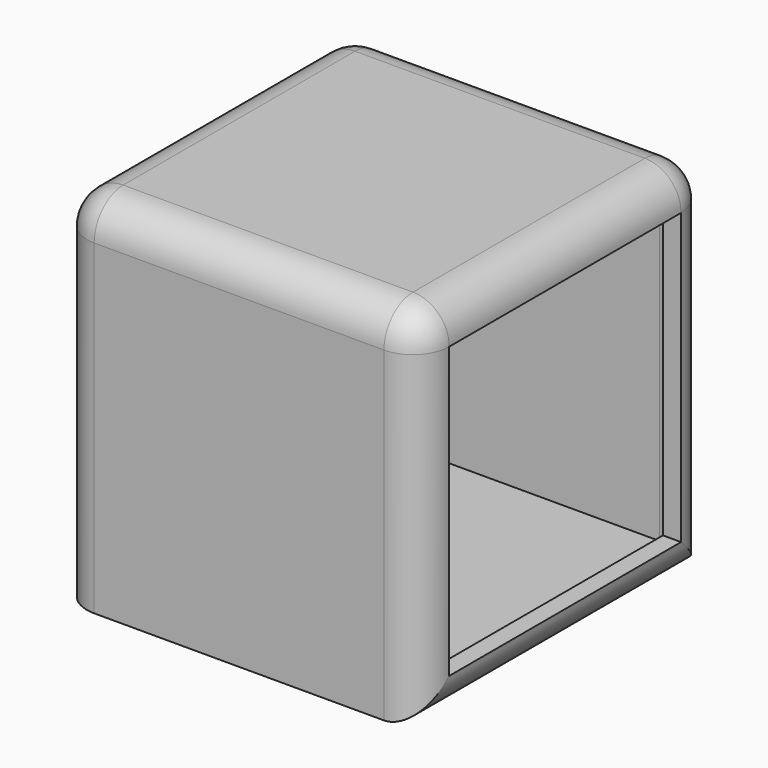
from build123d import *

# Parameters (mm, degrees)
F0_W     = 50.8
F0_H     = 50.8
F1_DEPTH = 50.8
F3_R     = 5.08
F4_T     = -2.54


# Not quite as in the source:
# - a shell that OpenCascade refuses in one call is made with other operations: the cavity is built on its own and cut out


with BuildPart() as f1:
    # F0 (on Top) → F1 (new body)
    with BuildSketch(Plane.XY):
        with Locations((-29.015717721, -32.2184429228)):
            Rectangle(F0_W, F0_H)
    extrude(amount=F1_DEPTH)

    # F3
    f3_edges = [f1.edges().sort_by_distance(p)[0] for p in [
        (-29.015718, -57.618443, 50.8),
        (-54.415718, -32.218443, 50.8),
        (-29.015718, -6.818443, 50.8),
        (-3.615718, -32.218443, 50.8),
        (-54.415718, -57.618443, 25.4),
        (-54.415718, -6.818443, 25.4),
        (-3.615718, -6.818443, 25.4),
        (-3.615718, -57.618443, 25.4),
        (-3.615718, -32.218443, 0),
    ]]
    fillet(f3_edges, radius=F3_R)

    # F4: a shell. OpenCascade refuses it in one call, so the cavity is built on its own and cut out:
    # the body offset inwards by the wall thickness, plus a prism from it out through each open face.
    f4_core = offset(f1.part, amount=F4_T, mode=Mode.PRIVATE)
    f4_exits = [f4_core.faces().sort_by_distance(p)[0] for p in [
        (-6.155718, -32.218443, 25.4),
    ]]
    add(f4_core, mode=Mode.SUBTRACT)
    extrude(f4_exits, amount=-F4_T, mode=Mode.SUBTRACT)


solid = f1.part
